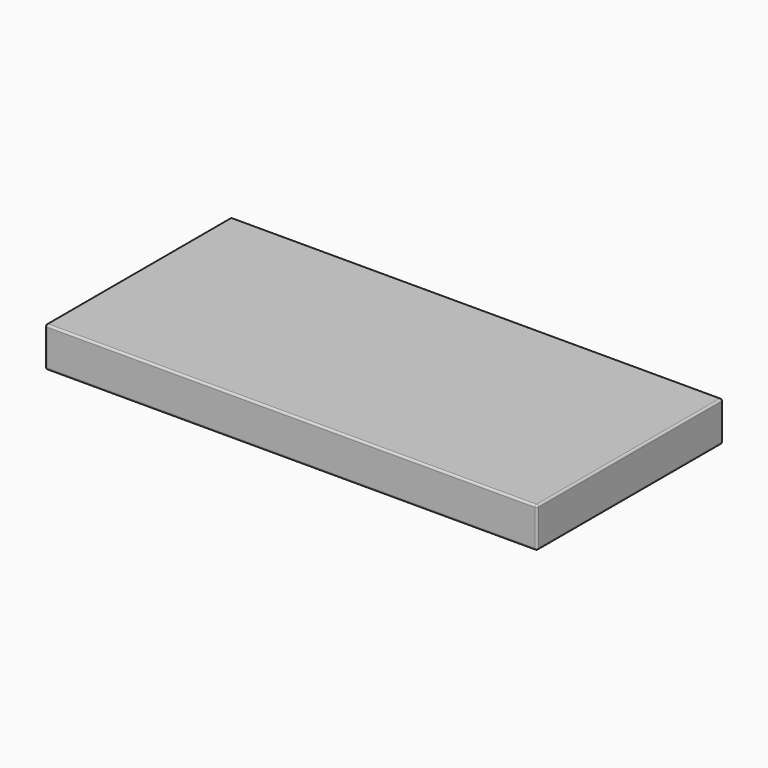
from build123d import *

# Parameters (mm, degrees)
F0_W         = 370
F0_H         = 175
F1_DEPTH     = 30
F2_T         = -4
F3_R         = 1.5
F4_T1_DEPTH  = 172
F4_T3_DEPTH  = 27
F4_T5_DEPTH  = 367
F4_S9_W      = 1.5
F4_S9_H      = 1.5
F4_T10_DEPTH = 1.5
F4_S15_W     = 1.5
F4_S15_H     = 1.5
F4_T16_DEPTH = 1.5
F4_S21_W     = 1.5
F4_S21_H     = 1.5
F4_T22_DEPTH = 1.5
F4_S27_W     = 1.5
F4_S27_H     = 1.5
F4_T28_DEPTH = 1.5
F4_S33_W     = 1.5
F4_S33_H     = 1.5
F4_T34_DEPTH = 1.5
F4_S39_W     = 1.5
F4_S39_H     = 1.5
F4_T40_DEPTH = 1.5
F4_S45_W     = 1.5
F4_S45_H     = 1.5
F4_T46_DEPTH = 1.5
F4_S51_W     = 1.5
F4_S51_H     = 1.5
F4_T52_DEPTH = 1.5


# Not quite as in the source:
# - a fillet or chamfer that OpenCascade refuses, or shapes differently, is made with other operations: its cross-section is extruded or revolved along the edge and cut away or added


with BuildPart() as f1:
    # F0 (on Top) → F1 (new body)
    with BuildSketch(Plane.XY):
        with Locations((128.3509446681, -49.7856229544)):
            Rectangle(F0_W, F0_H)
    extrude(amount=F1_DEPTH)

    # F2
    f2_openings = [f1.faces().sort_by_distance(p)[0] for p in [
        (128.350945, -49.785623, 0),
    ]]
    offset(amount=F2_T, openings=f2_openings)

    # F3
    f3_edges = [f1.edges().sort_by_distance(p)[0] for p in [
        (128.350945, -137.285623, 0),
        (-56.649055, -49.785623, 0),
        (-52.649055, -49.785623, 0),
        (128.350945, -133.285623, 0),
        (128.350945, 37.714377, 0),
        (128.350945, 33.714377, 0),
        (309.350945, -49.785623, 0),
        (313.350945, -49.785623, 0),
    ]]
    fillet(f3_edges, radius=F3_R)

    # F4: fillet of radius 1.5 on 8 edges, made by hand

    # F4_s2 → F4_t1 (cut)
    with BuildSketch(Plane.XZ.offset(-36.2143770456)):
        with BuildLine():
            ThreePointArc((-55.1490553319, 30), (-56.2097155037, 29.5606601718), (-56.6490553319, 28.5))
            Line((-56.6490553319, 28.5), (-56.6490553319, 30))
            Line((-56.6490553319, 30), (-55.1490553319, 30))
        make_face()
        with BuildLine():
            ThreePointArc((313.3509446681, 28.5), (312.9116048398, 29.5606601718), (311.8509446681, 30))
            Line((311.8509446681, 30), (313.3509446681, 30))
            Line((313.3509446681, 30), (313.3509446681, 28.5))
        make_face()
    extrude(amount=F4_T1_DEPTH, mode=Mode.SUBTRACT)

    # F4_s4 → F4_t3 (cut)
    with BuildSketch(Plane.XY.offset(1.5)):
        with BuildLine():
            ThreePointArc((-55.1490553319, 37.7143770456), (-56.2097155037, 37.2750372174), (-56.6490553319, 36.2143770456))
            Line((-56.6490553319, 36.2143770456), (-56.6490553319, 37.7143770456))
            Line((-56.6490553319, 37.7143770456), (-55.1490553319, 37.7143770456))
        make_face()
        with BuildLine():
            ThreePointArc((-56.6490553319, -135.7856229544), (-56.2097155037, -136.8462831261), (-55.1490553319, -137.2856229544))
            Line((-55.1490553319, -137.2856229544), (-56.6490553319, -137.2856229544))
            Line((-56.6490553319, -137.2856229544), (-56.6490553319, -135.7856229544))
        make_face()
        with BuildLine():
            ThreePointArc((313.3509446681, -135.7856229544), (312.9116048398, -136.8462831261), (311.8509446681, -137.2856229544))
            Line((311.8509446681, -137.2856229544), (313.3509446681, -137.2856229544))
            Line((313.3509446681, -137.2856229544), (313.3509446681, -135.7856229544))
        make_face()
        with BuildLine():
            ThreePointArc((311.8509446681, 37.7143770456), (312.9116048398, 37.2750372174), (313.3509446681, 36.2143770456))
            Line((313.3509446681, 36.2143770456), (313.3509446681, 37.7143770456))
            Line((313.3509446681, 37.7143770456), (311.8509446681, 37.7143770456))
        make_face()
    extrude(amount=F4_T3_DEPTH, mode=Mode.SUBTRACT)

    # F4_s6 → F4_t5 (cut)
    with BuildSketch(Plane.YZ.offset(-55.1490553319)):
        with BuildLine():
            ThreePointArc((-135.7856229544, 30), (-136.8462831261, 29.5606601718), (-137.2856229544, 28.5))
            Line((-137.2856229544, 28.5), (-137.2856229544, 30))
            Line((-137.2856229544, 30), (-135.7856229544, 30))
        make_face()
        with BuildLine():
            ThreePointArc((37.7143770456, 28.5), (37.2750372174, 29.5606601718), (36.2143770456, 30))
            Line((36.2143770456, 30), (37.7143770456, 30))
            Line((37.7143770456, 30), (37.7143770456, 28.5))
        make_face()
    extrude(amount=F4_T5_DEPTH, mode=Mode.SUBTRACT)


with BuildPart() as f4_tool8:
    # F4_s9 → F4_t10 (new body)
    with BuildSketch(Plane.XZ.offset(-36.2143770456)):
        with Locations((312.6009446681, 0.75)):
            Rectangle(F4_S9_W, F4_S9_H)
    extrude(amount=-F4_T10_DEPTH)

    # F4_s11 → F4_t12 (revolve, cut)
    with BuildSketch(Plane(origin=(311.8509446681, 36.2143770456, 1.5), x_dir=(-0.7071067812, 0, 0.7071067812), z_dir=(-0.7071067812, 0, -0.7071067812))):
        with BuildLine():
            ThreePointArc((0, -1.5), (1.5, 0), (0, 1.5))
            Line((0, 1.5), (0, -1.5))
        make_face()
    revolve(axis=Axis((311.8509446681, 36.2143770456, 1.5), (0, 1, 0)), mode=Mode.SUBTRACT)


with BuildPart() as f1_1:
    add(f1.part)

    # F4_t7: cut F4_tool8
    add(f4_tool8.part, mode=Mode.SUBTRACT)


with BuildPart() as f4_tool14:
    # F4_s15 → F4_t16 (new body)
    with BuildSketch(Plane.YZ.offset(311.8509446681)):
        with Locations((-136.5356229544, 0.75)):
            Rectangle(F4_S15_W, F4_S15_H)
    extrude(amount=F4_T16_DEPTH)

    # F4_s17 → F4_t18 (revolve, cut)
    with BuildSketch(Plane(origin=(311.8509446681, -135.7856229544, 1.5), x_dir=(0, 0.7071067812, 0.7071067812), z_dir=(0, 0.7071067812, -0.7071067812))):
        with BuildLine():
            ThreePointArc((0, -1.5), (1.5, 0), (0, 1.5))
            Line((0, 1.5), (0, -1.5))
        make_face()
    revolve(axis=Axis((311.8509446681, -135.7856229544, 1.5), (1, 0, 0)), mode=Mode.SUBTRACT)


with BuildPart() as f1_2:
    add(f1_1.part)

    # F4_t13: cut F4_tool14
    add(f4_tool14.part, mode=Mode.SUBTRACT)


with BuildPart() as f4_tool20:
    # F4_s21 → F4_t22 (new body)
    with BuildSketch(Plane.YZ.offset(-55.1490553319)):
        with Locations((-136.5356229544, 0.75)):
            Rectangle(F4_S21_W, F4_S21_H)
    extrude(amount=-F4_T22_DEPTH)

    # F4_s23 → F4_t24 (revolve, cut)
    with BuildSketch(Plane(origin=(-55.1490553319, -135.7856229544, 1.5), x_dir=(0, 0.7071067812, 0.7071067812), z_dir=(0, -0.7071067812, 0.7071067812))):
        with BuildLine():
            ThreePointArc((0, -1.5), (1.5, 0), (0, 1.5))
            Line((0, 1.5), (0, -1.5))
        make_face()
    revolve(axis=Axis((-55.1490553319, -135.7856229544, 1.5), (-1, 0, 0)), mode=Mode.SUBTRACT)


with BuildPart() as f1_3:
    add(f1_2.part)

    # F4_t19: cut F4_tool20
    add(f4_tool20.part, mode=Mode.SUBTRACT)


with BuildPart() as f4_tool26:
    # F4_s27 → F4_t28 (new body)
    with BuildSketch(Plane.XZ.offset(-36.2143770456)):
        with Locations((-55.8990553319, 0.75)):
            Rectangle(F4_S27_W, F4_S27_H)
    extrude(amount=-F4_T28_DEPTH)

    # F4_s29 → F4_t30 (revolve, cut)
    with BuildSketch(Plane(origin=(-55.1490553319, 36.2143770456, 1.5), x_dir=(0.7071067812, 0, 0.7071067812), z_dir=(-0.7071067812, 0, 0.7071067812))):
        with BuildLine():
            ThreePointArc((0, -1.5), (1.5, 0), (0, 1.5))
            Line((0, 1.5), (0, -1.5))
        make_face()
    revolve(axis=Axis((-55.1490553319, 36.2143770456, 1.5), (0, 1, 0)), mode=Mode.SUBTRACT)


with BuildPart() as f1_4:
    add(f1_3.part)

    # F4_t25: cut F4_tool26
    add(f4_tool26.part, mode=Mode.SUBTRACT)


with BuildPart() as f4_tool32:
    # F4_s33 → F4_t34 (new body)
    with BuildSketch(Plane.XZ.offset(-36.2143770456)):
        with Locations((-55.8990553319, 29.25)):
            Rectangle(F4_S33_W, F4_S33_H)
    extrude(amount=-F4_T34_DEPTH)

    # F4_s35 → F4_t36 (revolve, cut)
    with BuildSketch(Plane(origin=(-55.1490553319, 36.2143770456, 28.5), x_dir=(0.7071067812, 0, -0.7071067812), z_dir=(0.7071067812, 0, 0.7071067812))):
        with BuildLine():
            ThreePointArc((0, -1.5), (1.5, 0), (0, 1.5))
            Line((0, 1.5), (0, -1.5))
        make_face()
    revolve(axis=Axis((-55.1490553319, 36.2143770456, 28.5), (0, 1, 0)), mode=Mode.SUBTRACT)


with BuildPart() as f1_5:
    add(f1_4.part)

    # F4_t31: cut F4_tool32
    add(f4_tool32.part, mode=Mode.SUBTRACT)


with BuildPart() as f4_tool38:
    # F4_s39 → F4_t40 (new body)
    with BuildSketch(Plane.XY.offset(28.5)):
        with Locations((-55.8990553319, -136.5356229544)):
            Rectangle(F4_S39_W, F4_S39_H)
    extrude(amount=F4_T40_DEPTH)

    # F4_s41 → F4_t42 (revolve, cut)
    with BuildSketch(Plane(origin=(-55.1490553319, -135.7856229544, 28.5), x_dir=(0.7071067812, 0.7071067812, 0), z_dir=(0.7071067812, -0.7071067812, 0))):
        with BuildLine():
            ThreePointArc((0, -1.5), (1.5, 0), (0, 1.5))
            Line((0, 1.5), (0, -1.5))
        make_face()
    revolve(axis=Axis((-55.1490553319, -135.7856229544, 28.5), (0, 0, 1)), mode=Mode.SUBTRACT)


with BuildPart() as f1_6:
    add(f1_5.part)

    # F4_t37: cut F4_tool38
    add(f4_tool38.part, mode=Mode.SUBTRACT)


with BuildPart() as f4_tool44:
    # F4_s45 → F4_t46 (new body)
    with BuildSketch(Plane.YZ.offset(311.8509446681)):
        with Locations((-136.5356229544, 29.25)):
            Rectangle(F4_S45_W, F4_S45_H)
    extrude(amount=F4_T46_DEPTH)

    # F4_s47 → F4_t48 (revolve, cut)
    with BuildSketch(Plane(origin=(311.8509446681, -135.7856229544, 28.5), x_dir=(0, 0.7071067812, -0.7071067812), z_dir=(0, -0.7071067812, -0.7071067812))):
        with BuildLine():
            ThreePointArc((0, -1.5), (1.5, 0), (0, 1.5))
            Line((0, 1.5), (0, -1.5))
        make_face()
    revolve(axis=Axis((311.8509446681, -135.7856229544, 28.5), (1, 0, 0)), mode=Mode.SUBTRACT)


with BuildPart() as f1_7:
    add(f1_6.part)

    # F4_t43: cut F4_tool44
    add(f4_tool44.part, mode=Mode.SUBTRACT)


with BuildPart() as f4_tool50:
    # F4_s51 → F4_t52 (new body)
    with BuildSketch(Plane.XZ.offset(-36.2143770456)):
        with Locations((312.6009446681, 29.25)):
            Rectangle(F4_S51_W, F4_S51_H)
    extrude(amount=-F4_T52_DEPTH)

    # F4_s53 → F4_t54 (revolve, cut)
    with BuildSketch(Plane(origin=(311.8509446681, 36.2143770456, 28.5), x_dir=(-0.7071067812, 0, -0.7071067812), z_dir=(0.7071067812, 0, -0.7071067812))):
        with BuildLine():
            ThreePointArc((0, -1.5), (1.5, 0), (0, 1.5))
            Line((0, 1.5), (0, -1.5))
        make_face()
    revolve(axis=Axis((311.8509446681, 36.2143770456, 28.5), (0, 1, 0)), mode=Mode.SUBTRACT)


with BuildPart() as f1_8:
    add(f1_7.part)

    # F4_t49: cut F4_tool50
    add(f4_tool50.part, mode=Mode.SUBTRACT)


solid = f1_8.part
